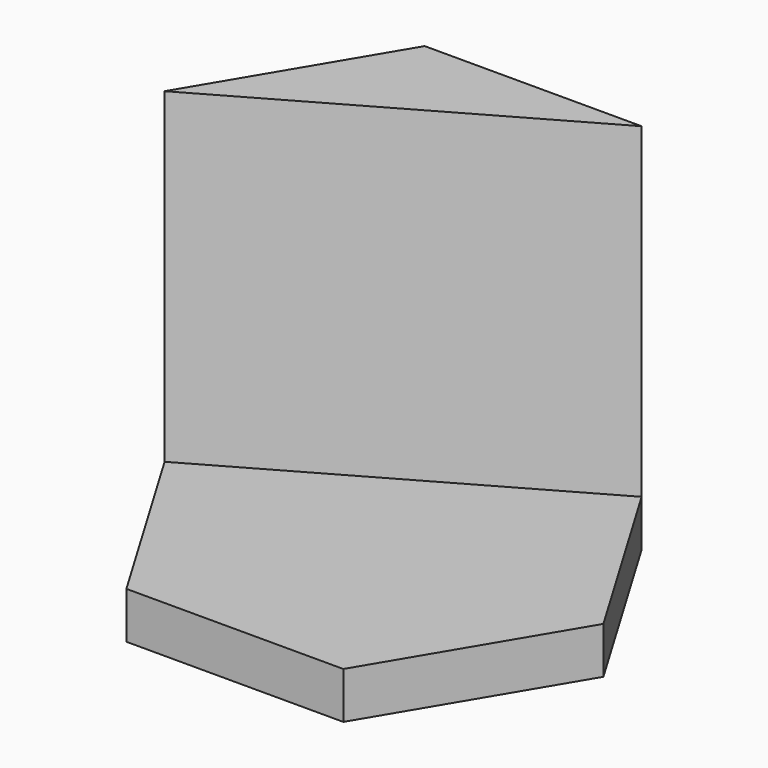
from build123d import *

# Parameters (mm, degrees)
F1_DEPTH = 3.175
F3_DEPTH = 22.225


# Not quite as in the source:
# - a feature names something its author has since deleted; it is built from what else it names


with BuildPart() as f1:
    # F0 (on Top) → F1 (new body)
    with BuildSketch(Plane.XY):
        Polygon((7.557114383, 12.7), (0, 0), (7.557114383, -12.7), (22.3354761934, -12.7), (29.8925905764, 0), (22.3354761934, 12.7), align=None)
    extrude(amount=F1_DEPTH)

    # F2 (on face) → F3 (join)
    with BuildSketch(Plane.XY.offset(3.175)):
        Polygon((7.557114383, 12.7), (0, 0), (22.3354761934, 12.7), align=None)
    extrude(amount=F3_DEPTH)


solid = f1.part
